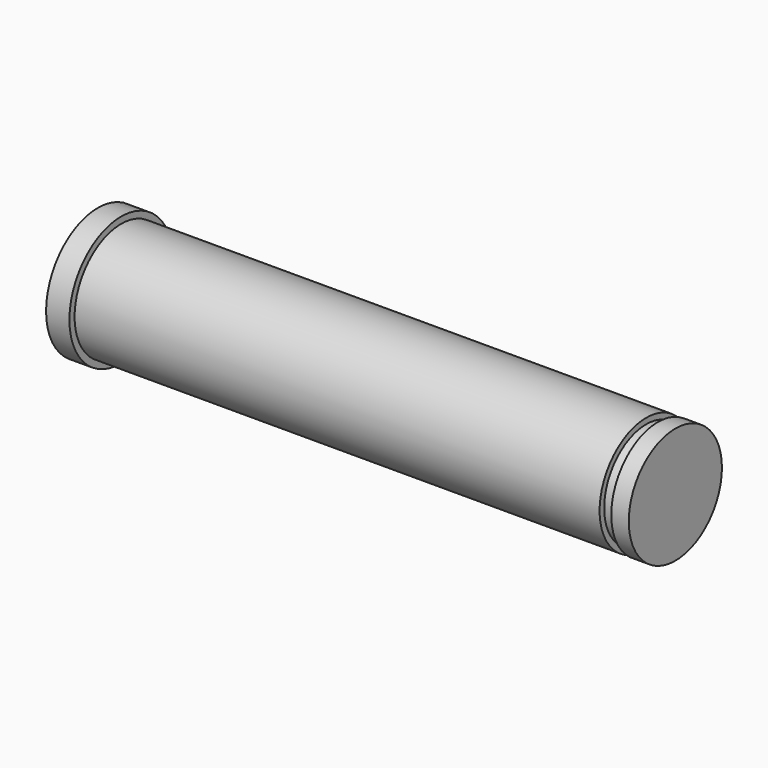
from build123d import *

# Parameters (mm, degrees)
F0_R     = 4.99
F1_DEPTH = 45
F2_R     = 5.5454073787
F2_R_2   = 4.99
F3_DEPTH = 2
F4_R     = 4.5
F5_DEPTH = 1
F6_R     = 4.99
F6_R_2   = 4.5
F7_DEPTH = 1.5


with BuildPart() as f1:
    # F0 (on Right) → F1 (new body)
    with BuildSketch(Plane.YZ):
        Circle(F0_R)
    extrude(amount=F1_DEPTH)

    # F2 (on face) → F3 (join)
    with BuildSketch(Plane(origin=(0, 0, 0), x_dir=(0, -1, 0), z_dir=(-1, 0, 0))):
        Circle(F2_R)
        Circle(F2_R_2, mode=Mode.SUBTRACT)
        Circle(F2_R_2)
    extrude(amount=F3_DEPTH)

    # F4 (on face) → F5 (join)
    with BuildSketch(Plane.YZ.offset(45)):
        Circle(F4_R)
    extrude(amount=F5_DEPTH)

    # F6 (on face) → F7 (join)
    with BuildSketch(Plane.YZ.offset(46)):
        Circle(F6_R)
        Circle(F6_R_2, mode=Mode.SUBTRACT)
        Circle(F6_R_2)
    extrude(amount=F7_DEPTH)


solid = f1.part
